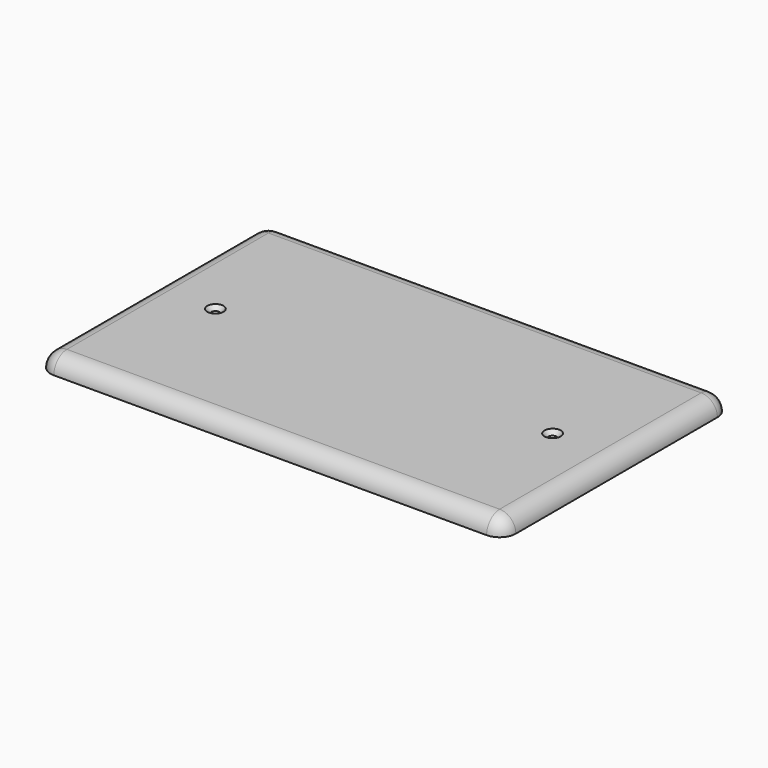
from build123d import *

# Parameters (mm, degrees)
F0_W           = 114.5
F0_H           = 70
F1_DEPTH       = 4
F2_R           = 3.99999
F3_T           = -1
F5_D           = 2
F5_CSINK_D     = 4
F5_CSINK_ANGLE = 90


# Not quite as in the source:
# - a fillet or chamfer is up to 0.001 mm smaller than in the source, because OpenCascade refuses the exact size


with BuildPart() as f1:
    # F0 (on Top) → F1 (new body)
    with BuildSketch(Plane.XY):
        Rectangle(F0_W, F0_H)
    extrude(amount=F1_DEPTH)

    # F2 (radius 4 in the source; OpenCascade refuses exactly that, so slightly less here)
    f2_edges = [f1.edges().sort_by_distance(p)[0] for p in [
        (-57.25, 0, 4),
        (0, 35, 4),
        (0, -35, 4),
        (-57.25, -35, 2),
        (-57.25, 35, 2),
        (57.25, 35, 2),
        (57.25, 0, 4),
        (57.25, -35, 2),
    ]]
    fillet(f2_edges, radius=F2_R)

    # F3
    f3_openings = [f1.faces().sort_by_distance(p)[0] for p in [
        (0, 0, 0),
    ]]
    offset(amount=F3_T, openings=f3_openings)

    # F5 (through all)
    with Locations(Plane.XY.offset(4)):
        with Locations((41.5, 0), (-41.5, 0)):
            CounterSinkHole(F5_D / 2, F5_CSINK_D / 2, counter_sink_angle=F5_CSINK_ANGLE)


solid = f1.part
